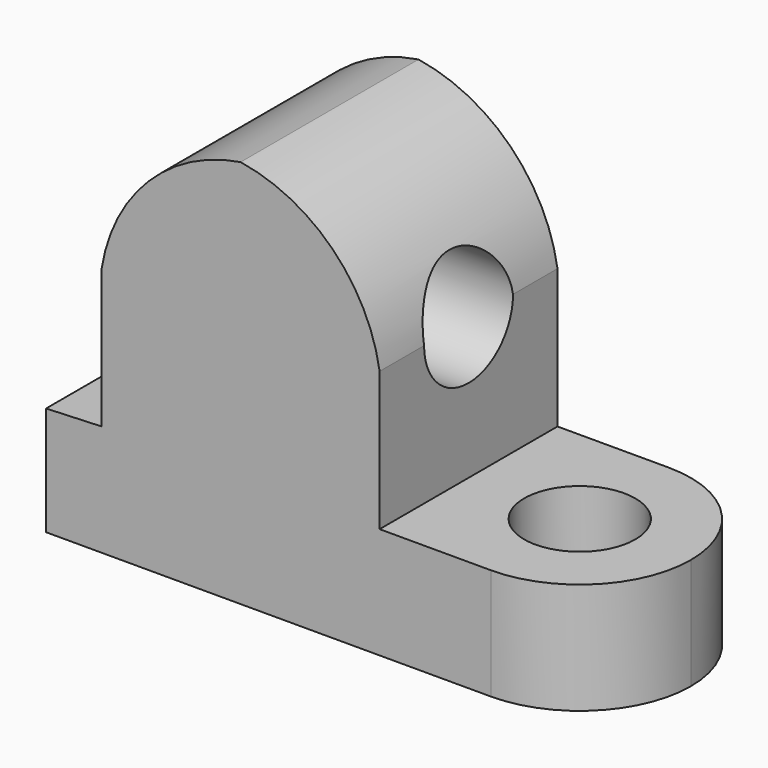
from build123d import *

# Parameters (mm, degrees)
F1_DEPTH = 25.4
F3_DEPTH = 25.4
F4_R     = 6.35
F5_DEPTH = 25.4
F7_DEPTH = 25.4
F9_DEPTH = 25.4


# Not quite as in the source:
# - ends of sketch curves that miss each other by under 0.0002 mm in the source are joined


with BuildPart() as f1:
    # F0 (on Front) → F1 (new body)
    with BuildSketch(Plane.XZ):
        Polygon((-67.7254482706, 28.6358930171), (-67.7254482706, 16.1884303746), (-4.2254482706, 16.1884303746), (-4.2254482706, 28.8884303746), (-29.6254482706, 28.8884303746), (-29.6254482706, 60.6384303746), (-61.3754482706, 60.6384303746), (-61.3754482706, 28.8884303746), align=None)
    extrude(amount=F1_DEPTH)

    # F2 (on face) → F3 (cut)
    with BuildSketch(Plane.XY.offset(28.8884303746)):
        with BuildLine():
            ThreePointArc((-16.9254482706, 0), (-7.9451915343, -3.7197435424), (-4.2254473189, -12.7))
            Line((-4.2254473189, -12.7), (-4.2254482706, 0))
            Line((-4.2254482706, 0), (-16.9254482706, 0))
        make_face()
        with BuildLine():
            ThreePointArc((-4.2254473189, -12.7), (-7.9451908613, -21.6802557846), (-16.9254463672, -25.4))
            Line((-16.9254463672, -25.4), (-4.2254482706, -25.4))
            Line((-4.2254482706, -25.4), (-4.2254473189, -12.7))
        make_face()
    extrude(amount=-F3_DEPTH, mode=Mode.SUBTRACT)

    # F4 (on face) → F5 (cut)
    with BuildSketch(Plane.XY.offset(28.8884303746)):
        with Locations((-16.9254473189, -12.7)):
            Circle(F4_R)
    extrude(amount=-F5_DEPTH, mode=Mode.SUBTRACT)

    # F6 (on face) → F7 (cut)
    with BuildSketch(Plane.XZ.offset(25.4)):
        with BuildLine():
            ThreePointArc((-45.5004482706, 60.6384303746), (-34.9759157672, 55.287962878), (-29.6254482706, 44.7634303746))
            Line((-29.6254482706, 44.7634303746), (-29.6254482706, 60.6384303746))
            Line((-29.6254482706, 60.6384303746), (-45.5004482706, 60.6384303746))
        make_face()
        with BuildLine():
            ThreePointArc((-61.3754482706, 44.7634303746), (-56.0249807741, 55.287962878), (-45.5004482706, 60.6384303746))
            Line((-45.5004482706, 60.6384303746), (-61.3754482706, 60.6384303746))
            Line((-61.3754482706, 60.6384303746), (-61.3754482706, 44.7634303746))
        make_face()
    extrude(amount=-F7_DEPTH, mode=Mode.SUBTRACT)

    # F8 (on face) → F9 (cut)
    with BuildSketch(Plane.YZ.offset(-29.6254482706)):
        with BuildLine():
            ThreePointArc((-19.05, 44.7634303746), (-12.7, 38.4134303746), (-6.35, 44.7634303746))
            Line((-6.35, 44.7634303746), (-19.05, 44.7634303746))
        make_face()
        with BuildLine():
            Line((-19.05, 44.7634303746), (-6.35, 44.7634303746))
            ThreePointArc((-6.35, 44.7634303746), (-12.7, 51.1134303746), (-19.05, 44.7634303746))
        make_face()
    extrude(amount=-F9_DEPTH, mode=Mode.SUBTRACT)


solid = f1.part
